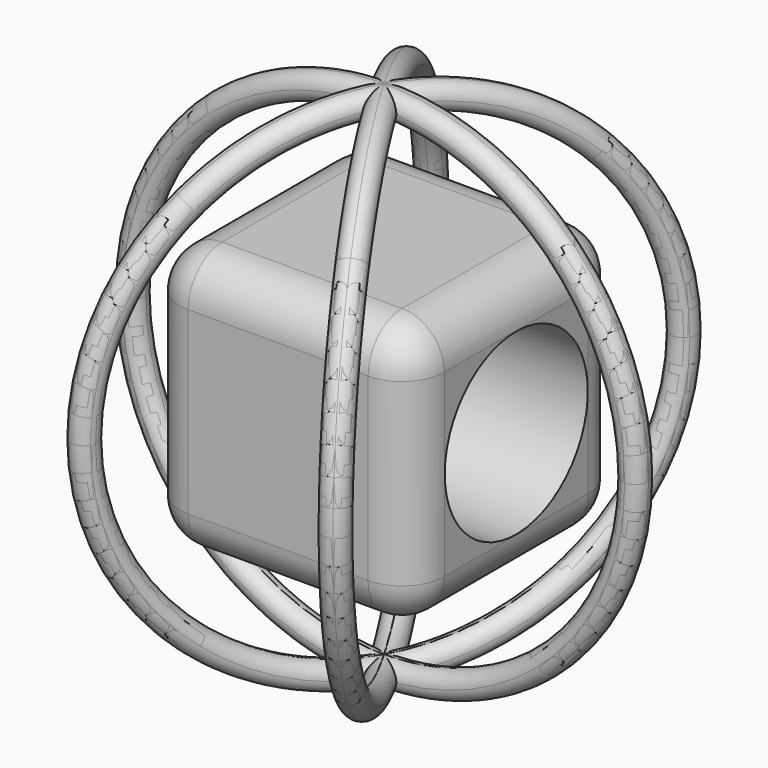
from build123d import *

# Parameters (mm, degrees)
F0_W          = 50
F0_H          = 50
F1_DEPTH      = 25
F1_DEPTH_BACK = 25
F2_R          = 50
F2_R_2        = 45.0000017881
F3_DEPTH      = 2.5
F3_DEPTH_BACK = 2.5
F4_R          = 2.49999
F6_COUNT      = 6
F7_R          = 8
F8_R          = 16.895
F9_DEPTH      = 50


# Not quite as in the source:
# - a fillet or chamfer is up to 0.001 mm smaller than in the source, because OpenCascade refuses the exact size


with BuildPart() as f1:
    # F0 (on Top) → F1 (new body, two sides)
    with BuildSketch(Plane.XY) as f1_sk:
        Rectangle(F0_W, F0_H)
    extrude(amount=F1_DEPTH)
    extrude(f1_sk.sketch, amount=-F1_DEPTH_BACK)

    # F7
    f7_edges = [f1.edges().sort_by_distance(p)[0] for p in [
        (0, -25, 25),
        (-25, 0, 25),
        (0, 25, 25),
        (-25, 0, -25),
        (-25, -25, 0),
        (0, -25, -25),
        (25, -25, 0),
        (25, 0, 25),
        (25, 0, -25),
        (25, 25, 0),
        (0, 25, -25),
        (-25, 25, 0),
    ]]
    fillet(f7_edges, radius=F7_R)

    # F8 (on face) → F9 (cut)
    with BuildSketch(Plane(origin=(-25, 0, 0), x_dir=(0, -1, 0), z_dir=(-1, 0, 0))):
        Circle(F8_R)
    extrude(amount=-F9_DEPTH, mode=Mode.SUBTRACT)


with BuildPart() as f3:
    # F2 (on Front) → F3 (new body, two sides)
    with BuildSketch(Plane.XZ) as f3_sk:
        Circle(F2_R)
        Circle(F2_R_2, mode=Mode.SUBTRACT)
    extrude(amount=F3_DEPTH)
    extrude(f3_sk.sketch, amount=-F3_DEPTH_BACK)

    # F4 (radius 2.5 in the source; OpenCascade refuses exactly that, so slightly less here)
    f4_edges = [f3.edges().sort_by_distance(p)[0] for p in [
        (-50, -2.5, 0),
        (-45.000002, -2.5, 0),
        (50, 1.25, 0),
        (-50, 0, 0),
        (-50, 2.5, 0),
        (-45.000002, 2.5, 0),
    ]]
    fillet(f4_edges, radius=F4_R)


with BuildPart() as f6_1:
    # F6: instance of F3
    add(f3.part.rotate(Axis((0, 0, 0), (0, 0, 1)), 1 * 360 / F6_COUNT))


with BuildPart() as f6_2:
    # F6: instance of F3
    add(f3.part.rotate(Axis((0, 0, 0), (0, 0, 1)), 2 * 360 / F6_COUNT))


with BuildPart() as f6_3:
    # F6: instance of F3
    add(f3.part.rotate(Axis((0, 0, 0), (0, 0, 1)), 3 * 360 / F6_COUNT))


with BuildPart() as f6_4:
    # F6: instance of F3
    add(f3.part.rotate(Axis((0, 0, 0), (0, 0, 1)), 4 * 360 / F6_COUNT))


with BuildPart() as f6_5:
    # F6: instance of F3
    add(f3.part.rotate(Axis((0, 0, 0), (0, 0, 1)), 5 * 360 / F6_COUNT))


solid = Compound([f1.part, f3.part, f6_1.part, f6_2.part, f6_3.part, f6_4.part, f6_5.part])
